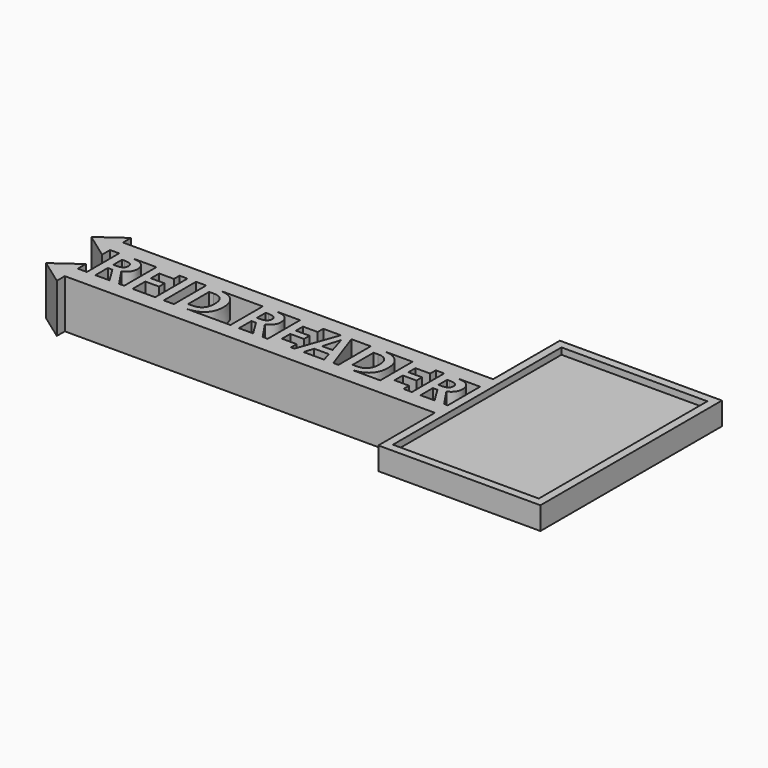
from build123d import *

# Parameters (mm, degrees)
F0_TEXT_SIZE  = 17.4403984653
F1_DEPTH      = 5
F3_DEPTH      = 15
F4_W          = 50
F4_H          = 70
F5_DEPTH      = 5
F5_DEPTH_BACK = 2
F6_W          = 45
F6_H          = 65
F7_DEPTH      = 2


# Not quite as in the source:
# - Text() gives the source's letters only with a copy of the font that has no kerning and outlines rounded to 1/6400 em; it was checked with that copy


with BuildPart() as f1:
    # F0 (on Top) → F1 (new body)
    with BuildSketch(Plane.XY):
        with Locations((-112.9402053744, 0)):
            Text('RFID READER', F0_TEXT_SIZE, font='Open Sans', font_style=FontStyle.BOLD, text_align=(TextAlign.LEFT, TextAlign.BOTTOM))
    extrude(amount=F1_DEPTH)

    # F2 (on face) → F3 (join)
    with BuildSketch(Plane.XY.offset(5)):
        Polygon((-114.1627803445, 12.4508094669), (-111.3732945748, 12.4508094669), (0, 12.4508094669), (6.1189520347, 12.4508094669), (6.1189520347, 17.4508094669), (-111.3732945748, 17.4508094669), (-114.1627803445, 17.4508094669), (-114.1627803445, 20.5345991999), (-121.9448372722, 14.9508094669), (-114.1627803445, 9.3670197339), align=None)
        Polygon((-114.1627803445, 3.083789733), (-121.9448372722, -2.5), (-114.1627803445, -8.083789733), (-114.1627803445, -5), (6.1189520347, -5), (6.1189520347, 0), (0, 0), (-111.3732945748, 0), (-114.1627803445, 0), align=None)
    extrude(amount=-F3_DEPTH)

    # F4 (on Top) → F5 (join, two sides)
    with BuildSketch(Plane.XY) as f5_sk:
        with Locations((25, 8.2128791511)):
            Rectangle(F4_W, F4_H)
    extrude(amount=F5_DEPTH)
    extrude(f5_sk.sketch, amount=-F5_DEPTH_BACK)

    # F6 (on face) → F7 (cut)
    with BuildSketch(Plane.XY.offset(5)):
        with Locations((25, 8.2128791511)):
            Rectangle(F6_W, F6_H)
    extrude(amount=-F7_DEPTH, mode=Mode.SUBTRACT)


solid = f1.part
